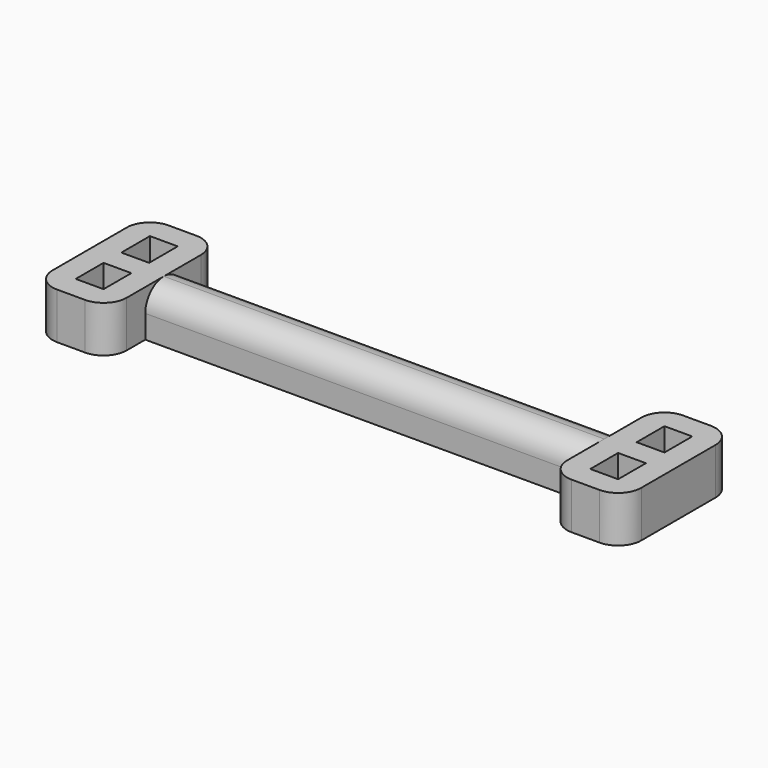
from build123d import *

# Parameters (mm, degrees)
F0_W     = 6
F0_H     = 7.5
F0_H_2   = 7.7
F1_DEPTH = 10
F0_W_2   = 95
F0_H_3   = 10
F2_DEPTH = 10
F3_R     = 4.99999
F4_R     = 5


# Not quite as in the source:
# - a fillet or chamfer is up to 0.001 mm smaller than in the source, because OpenCascade refuses the exact size


with BuildPart() as f1:
    # F0 (on Top) → F1 (new body)
    with BuildSketch(Plane.XY):
        Polygon((-46.5609904528, 20.46333462), (-46.5609904528, 30.46333462), (-46.5609904528, 40.46333462), (-62.5609904528, 40.46333462), (-62.5609904528, 10.46333462), (-46.5609904528, 10.46333462), align=None)
        with Locations((-54.5609904528, 19.21333462)):
            Rectangle(F0_W, F0_H, mode=Mode.SUBTRACT)
        with Locations((-54.5609904528, 31.61333462)):
            Rectangle(F0_W, F0_H_2, mode=Mode.SUBTRACT)
    extrude(amount=F1_DEPTH)



with BuildPart() as f1b:
    # F0 (on Top) → F1, piece 2 (new body)
    with BuildSketch(Plane.XY):
        Polygon((48.4390095472, 40.46333462), (48.4390095472, 30.46333462), (48.4390095472, 20.46333462), (48.4390095472, 10.46333462), (64.4390095472, 10.46333462), (64.4390095472, 40.46333462), align=None)
        with Locations((56.4390095472, 19.21333462)):
            Rectangle(F0_W, F0_H, mode=Mode.SUBTRACT)
        with Locations((56.4390095472, 31.71333462)):
            Rectangle(F0_W, F0_H, mode=Mode.SUBTRACT)
    extrude(amount=F1_DEPTH)


with BuildPart() as f1_1:
    add(f1.part)

    add(f1b.part)  # F2 merges F1b
    # F0 (on Top) → F2 (join)
    with BuildSketch(Plane.XY):
        with Locations((0.9390095472, 25.46333462)):
            Rectangle(F0_W_2, F0_H_3)
    extrude(amount=F2_DEPTH)

    # F3 (radius 5 in the source; OpenCascade refuses exactly that, so slightly less here)
    f3_edges = [f1_1.edges().sort_by_distance(p)[0] for p in [
        (0.93901, 20.463335, 10),
        (0.93901, 30.463335, 10),
    ]]
    fillet(f3_edges, radius=F3_R)

    # F4
    f4_edges = [f1_1.edges().sort_by_distance(p)[0] for p in [
        (-62.56099, 10.463335, 5),
        (-46.56099, 10.463335, 5),
        (48.43901, 10.463335, 5),
        (64.43901, 10.463335, 5),
        (64.43901, 40.463335, 5),
        (48.43901, 40.463335, 5),
        (-46.56099, 40.463335, 5),
        (-62.56099, 40.463335, 5),
    ]]
    fillet(f4_edges, radius=F4_R)


solid = f1_1.part
